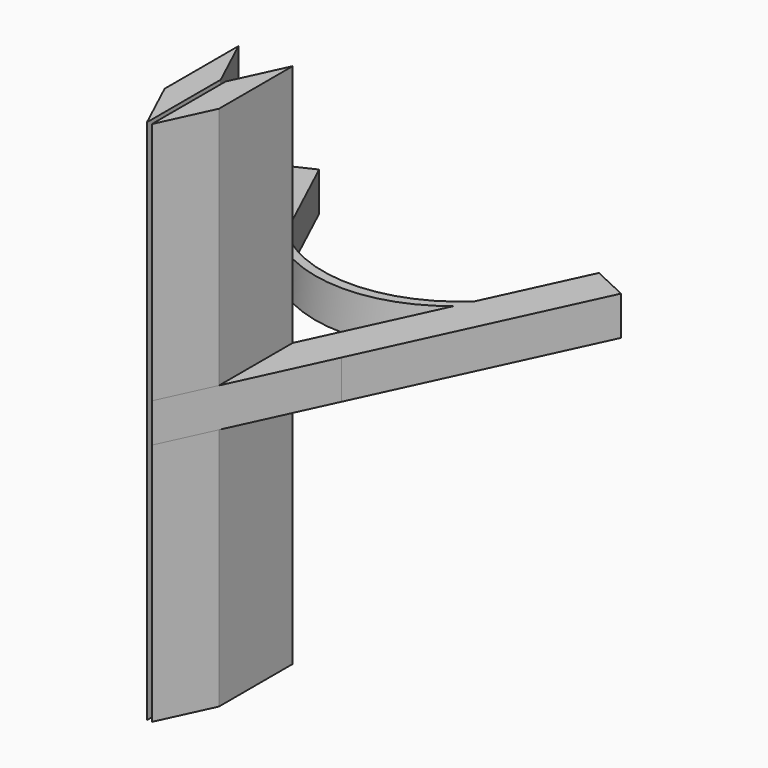
from build123d import *

# Parameters (mm, degrees)
F1_DEPTH  = 2
F3_DEPTH  = 4
F4_W      = 0.5
F4_H      = 15
F5_DEPTH  = 25
F6_DEPTH  = 2
F8_DEPTH  = 25
F10_DEPTH = 25


with BuildPart() as f1:
    # F0 (on Top) → F1 (new body)
    with BuildSketch(Plane.XY):
        Polygon((-7.4135116758, 0), (-0.25, -15.362200364), (-0.25, -5.8973940314), (-3, 0), (-14.3537370712, 24.3481677229), (-17.9789682194, 22.6576946759), align=None)
        Polygon((0.25, -15.362200364), (7.4135116758, 0), (17.9789682194, 22.6576946759), (14.3537370712, 24.3481677229), (3, 0), (0.25, -5.8973940314), align=None)
        Polygon((0, -15.8983270941), (0.25, -15.362200364), (0.25, -5.8973940314), (0, -6.4335207615), (-0.25, -5.8973940314), (-0.25, -15.362200364), align=None)
    extrude(amount=F1_DEPTH)

    # F2 (on face) → F3 (join)
    with BuildSketch(Plane.XY.offset(2)):
        with BuildLine():
            ThreePointArc((-8.8668911775, 12.581588732), (0, 9.4157126397), (8.8668911775, 12.581588732))
            Line((8.8668911775, 12.581588732), (9.6599709615, 14.2823538173))
            ThreePointArc((9.6599709615, 14.2823538173), (0, 10.4157126397), (-9.6599709615, 14.2823538173))
            Line((-9.6599709615, 14.2823538173), (-8.8668911775, 12.581588732))
        make_face()
        with BuildLine():
            ThreePointArc((-13.9989482009, 23.5873205351), (-12.6883090185, 17.4990569753), (-8.8668911775, 12.581588732))
            Line((-8.8668911775, 12.581588732), (-9.6599709615, 14.2823538173))
            ThreePointArc((-9.6599709615, 14.2823538173), (-12.6883090185, 18.4990569753), (-13.97191286, 23.5293430595))
            Line((-13.97191286, 23.5293430595), (-13.9989482009, 23.5873205351))
        make_face()
        with BuildLine():
            ThreePointArc((-13.97191286, 23.5293430595), (-12.6883090185, 18.4990569753), (-9.6599709615, 14.2823538173))
            Line((-9.6599709615, 14.2823538173), (-13.97191286, 23.5293430595))
        make_face()
    extrude(amount=-F3_DEPTH)

    # F4 (on face) → F5 (cut)
    with BuildSketch(Plane.XY.offset(2)):
        with Locations((0, -9.3687182158)):
            Rectangle(F4_W, F4_H)
    extrude(amount=-F5_DEPTH, mode=Mode.SUBTRACT)

    # F6 (add): faces of the model
    f6_faces = [f1.faces().sort_by_distance(p)[0] for p in [
        (-7.9421134858, 5.393960994, 0),
        (8.2425809304, 6.3306998172, 0),
    ]]
    extrude(f6_faces, amount=F6_DEPTH)

    # F7 (on face) → F8 (join)
    with BuildSketch(Plane.XY.offset(2)):
        Polygon((-0.25, -5.8973940314), (-2.7857095704, -0.4595473092), (-2.7857095704, -9.9243536418), (-0.25, -15.362200364), align=None)
        Polygon((2.7857095704, -9.9243536418), (2.7857095704, -0.4595473092), (0.25, -5.8973940314), (0.25, -15.362200364), align=None)
    extrude(amount=F8_DEPTH)

    # F9 (on face) → F10 (join)
    with BuildSketch(Plane(origin=(0, 0, -2), x_dir=(1, 0, 0), z_dir=(0, 0, -1))):
        Polygon((-0.25, 15.362200364), (-2.7857095704, 9.9243536418), (-2.7857095704, 0.4595473092), (-0.25, 5.8973940314), align=None)
        Polygon((0.25, 5.8973940314), (2.7857095704, 0.4595473092), (2.7857095704, 9.9243536418), (0.25, 15.362200364), align=None)
    extrude(amount=F10_DEPTH)


solid = f1.part
